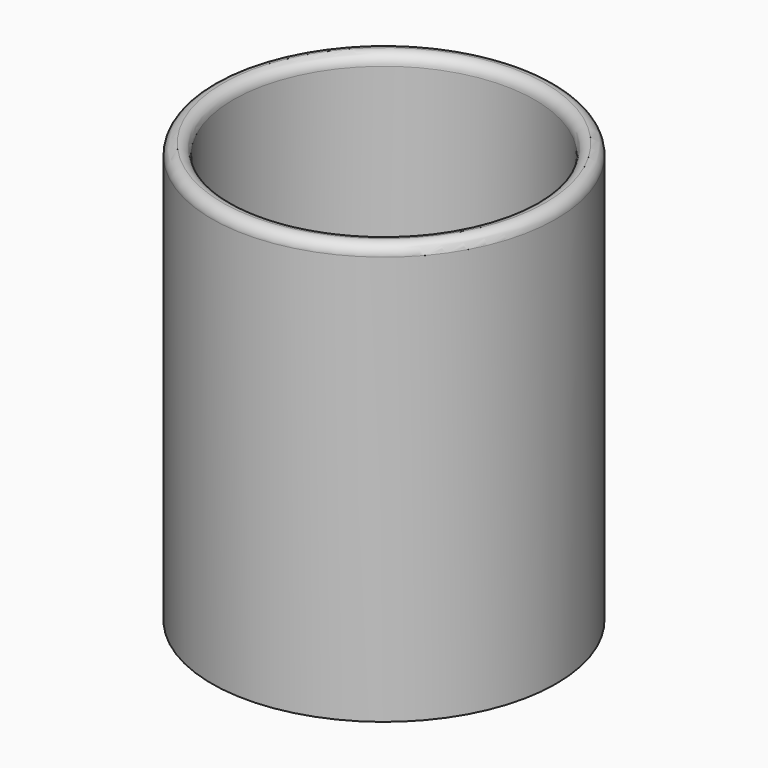
from build123d import *

# Parameters (mm, degrees)
F0_R     = 50.8
F0_R_2   = 44.45
F1_DEPTH = 123.825
F2_R     = 44.45
F3_DEPTH = 9.525
F4_R     = 3.17499


# Not quite as in the source:
# - a fillet or chamfer is up to 0.001 mm smaller than in the source, because OpenCascade refuses the exact size
# - a feature names something its author has since deleted; it is built from what else it names


with BuildPart() as f1:
    # F0 (on Top) → F1 (new body)
    with BuildSketch(Plane.XY):
        Circle(F0_R)
        Circle(F0_R_2, mode=Mode.SUBTRACT)
    extrude(amount=F1_DEPTH)

    # F2 (on Top) → F3 (join)
    with BuildSketch(Plane.XY):
        Circle(F2_R)
    extrude(amount=F3_DEPTH)

    # F4 (radius 3.175 in the source; OpenCascade refuses exactly that, so slightly less here)
    f4_edges = [f1.edges().sort_by_distance(p)[0] for p in [
        (-44.45, 0, 123.825),
        (-50.8, 0, 123.825),
    ]]
    fillet(f4_edges, radius=F4_R)


solid = f1.part
